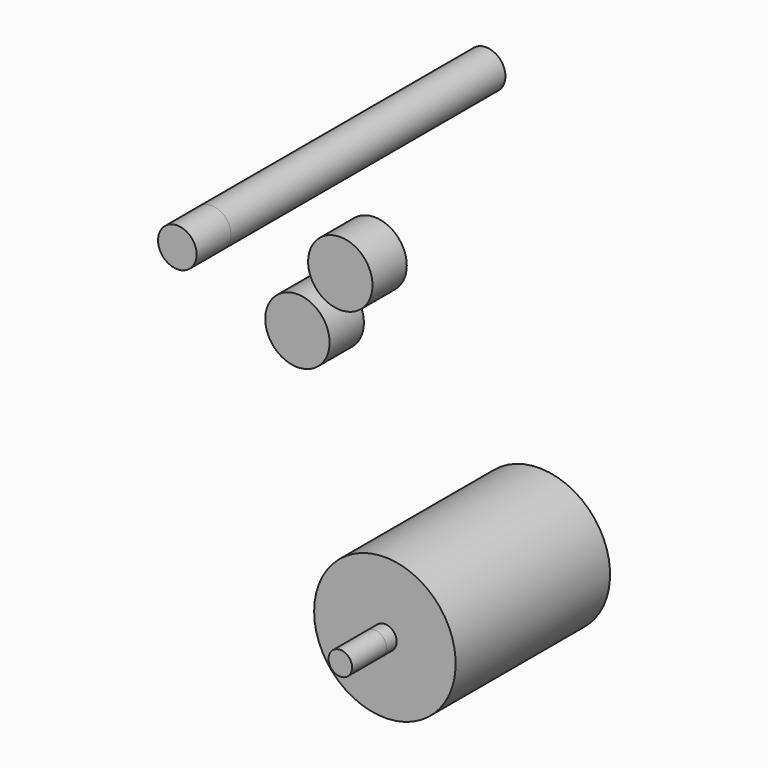
from build123d import *

# Parameters (mm, degrees)
F0_R     = 7.5
F1_DEPTH = 10
F0_R_2   = 4.5
F0_R_3   = 2.75
F3_R     = 4.5
F4_DEPTH = 80
F5_R     = 2.75
F6_DEPTH = 3
F7_R     = 16.5
F7_R_2   = 2.75
F8_DEPTH = 45


# Not quite as in the source:
# - the program builds the solid bodies; features that only make, move or delete a surface that nothing else refers to are left out


with BuildPart() as f1:
    # F0 (on Front) → F1 (new body)
    with BuildSketch(Plane.XZ):
        with Locations((0, 80)):
            Circle(F0_R)
    extrude(amount=F1_DEPTH)


with BuildPart() as f1b:
    # F0 (on Front) → F1, piece 2 (new body)
    with BuildSketch(Plane.XZ):
        with Locations((-38, 73)):
            Circle(F0_R_2)
    extrude(amount=F1_DEPTH)

    # F3 (on face) → F4 (join)
    with BuildSketch(Plane(origin=(0, 0, 0), x_dir=(-1, 0, 0), z_dir=(0, 1, 0))):
        with Locations((38, 73)):
            Circle(F3_R)
    extrude(amount=F4_DEPTH)


with BuildPart() as f1c:
    # F0 (on Front) → F1, piece 3 (new body)
    with BuildSketch(Plane.XZ):
        with Locations((-10, 65)):
            Circle(F0_R)
    extrude(amount=F1_DEPTH)


with BuildPart() as f1d:
    # F0 (on Front) → F1, piece 4 (new body)
    with BuildSketch(Plane.XZ):
        Circle(F0_R_3)
    extrude(amount=F1_DEPTH)

    # F5 (on face) → F6 (join)
    with BuildSketch(Plane(origin=(0, 0, 0), x_dir=(-1, 0, 0), z_dir=(0, 1, 0))):
        Circle(F5_R)
    extrude(amount=F6_DEPTH)


with BuildPart() as f8:
    # F7 (on face) → F8 (new body)
    with BuildSketch(Plane(origin=(0, 3, 0), x_dir=(-1, 0, 0), z_dir=(0, 1, 0))):
        Circle(F7_R)
        Circle(F7_R_2, mode=Mode.SUBTRACT)
    extrude(amount=F8_DEPTH)


solid = Compound([f1.part, f1b.part, f1c.part, f1d.part, f8.part])
